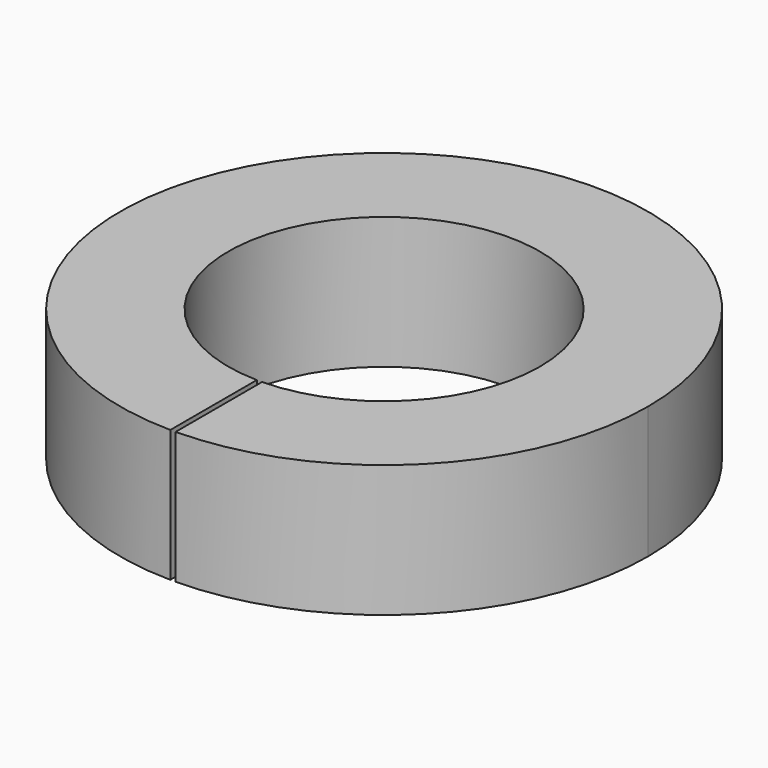
from build123d import *

# Parameters (mm, degrees)
F0_R     = 25.4
F0_R_2   = 15
F1_DEPTH = 6.35
F3_DEPTH = 12.701


with BuildPart() as f1:
    # F0 (on Top) → F1 (new body, symmetric)
    with BuildSketch(Plane.XY):
        Circle(F0_R)
        Circle(F0_R_2, mode=Mode.SUBTRACT)
    extrude(amount=F1_DEPTH, both=True)

    # F2 (on face) → F3 (cut, through all)
    with BuildSketch(Plane.XY.offset(6.35)):
        with BuildLine():
            ThreePointArc((0.254, -14.9978493125), (0, -15), (-0.254, -14.9978493125))
            Line((-0.254, -14.9978493125), (-0.254, -25.3987299682))
            ThreePointArc((-0.254, -25.3987299682), (0, -25.4), (0.254, -25.3987299682))
            Line((0.254, -25.3987299682), (0.254, -14.9978493125))
        make_face()
    extrude(amount=-F3_DEPTH, mode=Mode.SUBTRACT)


solid = f1.part
